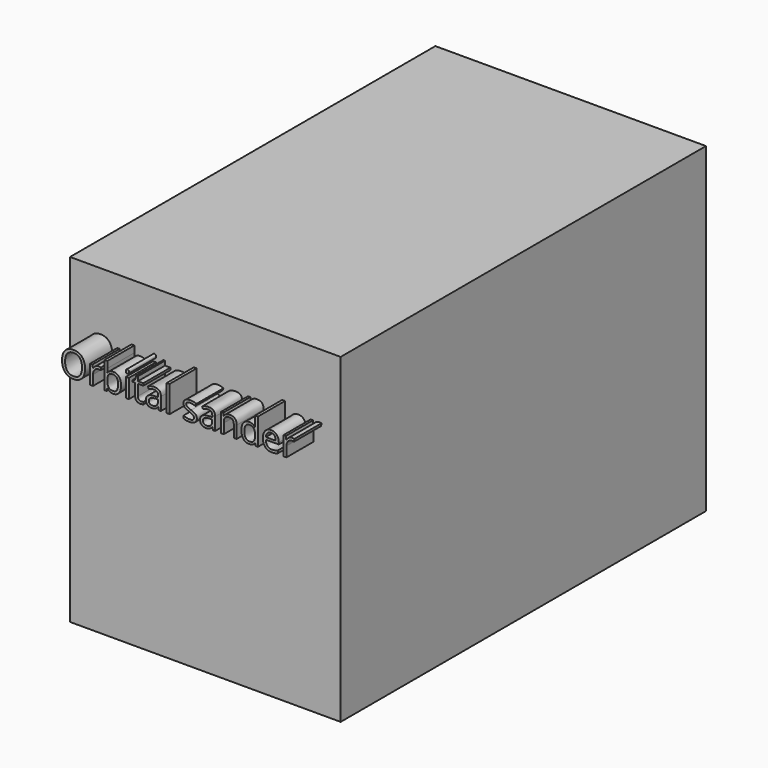
from build123d import *

# Parameters (mm, degrees)
F0_W         = 203.2
F0_H         = 241.3
F1_DEPTH     = 342.9
F2_TEXT_SIZE = 26.3236790969
F3_DEPTH     = 25.4


# Not quite as in the source:
# - Text() gives the source's letters only with a copy of the font that has no kerning and outlines rounded to 1/6400 em; it was checked with that copy


with BuildPart() as f1:
    # F0 (on Front) → F1 (new body)
    with BuildSketch(Plane.XZ):
        Rectangle(F0_W, F0_H)
    extrude(amount=F1_DEPTH)

    # F2 (on face) → F3 (join)
    with BuildSketch(Plane.XZ.offset(342.9)):
        with Locations((-88.9, 57.9118914313)):
            Text('Orbital sander', F2_TEXT_SIZE, font='Open Sans', text_align=(TextAlign.LEFT, TextAlign.BOTTOM))
    extrude(amount=F3_DEPTH)


solid = f1.part
